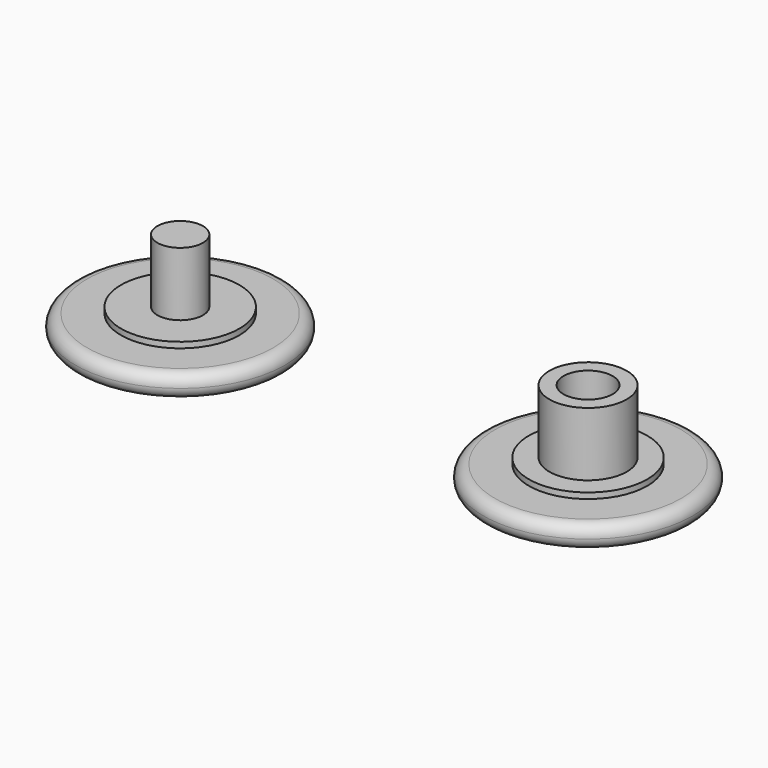
from build123d import *

# Parameters (mm, degrees)
F0_R      = 11.5
F0_R_2    = 6.5
F1_DEPTH  = 2.54
F0_R_3    = 4.25
F2_DEPTH  = 3.175
F3_DEPTH  = 10.175
F4_R      = 1.26999
F5_R      = 11.5
F5_R_2    = 6.5
F6_DEPTH  = 2.54
F5_R_3    = 2.5
F7_DEPTH  = 3.175
F8_DEPTH  = 10.175
F9_R      = 2.7
F10_DEPTH = 7
F11_R     = 1.26999


# Not quite as in the source:
# - a fillet or chamfer is up to 0.001 mm smaller than in the source, because OpenCascade refuses the exact size


with BuildPart() as f1:
    # F0 (on Top) → F1 (new body)
    with BuildSketch(Plane.XY):
        Circle(F0_R)
        Circle(F0_R_2, mode=Mode.SUBTRACT)
    extrude(amount=F1_DEPTH)

    # F0 (on Top) → F2 (join)
    with BuildSketch(Plane.XY):
        Circle(F0_R_2)
        Circle(F0_R_3, mode=Mode.SUBTRACT)
    extrude(amount=F2_DEPTH)

    # F0 (on Top) → F3 (join)
    with BuildSketch(Plane.XY):
        Circle(F0_R_3)
    extrude(amount=F3_DEPTH)

    # F4 (radius 1.27 in the source; OpenCascade refuses exactly that, so slightly less here)
    f4_edges = [f1.edges().sort_by_distance(p)[0] for p in [
        (-11.5, 0, 2.54),
        (-11.5, 0, 0),
    ]]
    fillet(f4_edges, radius=F4_R)

    # F9 (on face) → F10 (cut)
    with BuildSketch(Plane.XY.offset(10.175)):
        Circle(F9_R)
    extrude(amount=-F10_DEPTH, mode=Mode.SUBTRACT)


with BuildPart() as f6:
    # F5 (on Top) → F6 (new body)
    with BuildSketch(Plane.XY):
        with Locations((-44.7985892718, 0)):
            Circle(F5_R)
        with Locations((-44.7985892718, 0)):
            Circle(F5_R_2, mode=Mode.SUBTRACT)
    extrude(amount=F6_DEPTH)

    # F5 (on Top) → F7 (join)
    with BuildSketch(Plane.XY):
        with Locations((-44.7985892718, 0)):
            Circle(F5_R_2)
        with Locations((-44.7985892718, 0)):
            Circle(F5_R_3, mode=Mode.SUBTRACT)
    extrude(amount=F7_DEPTH)

    # F5 (on Top) → F8 (join)
    with BuildSketch(Plane.XY):
        with Locations((-44.7985892718, 0)):
            Circle(F5_R_3)
    extrude(amount=F8_DEPTH)

    # F11 (radius 1.27 in the source; OpenCascade refuses exactly that, so slightly less here)
    f11_edges = [f6.edges().sort_by_distance(p)[0] for p in [
        (-56.298589, 0, 2.54),
        (-56.298589, 0, 0),
    ]]
    fillet(f11_edges, radius=F11_R)


solid = Compound([f1.part, f6.part])
